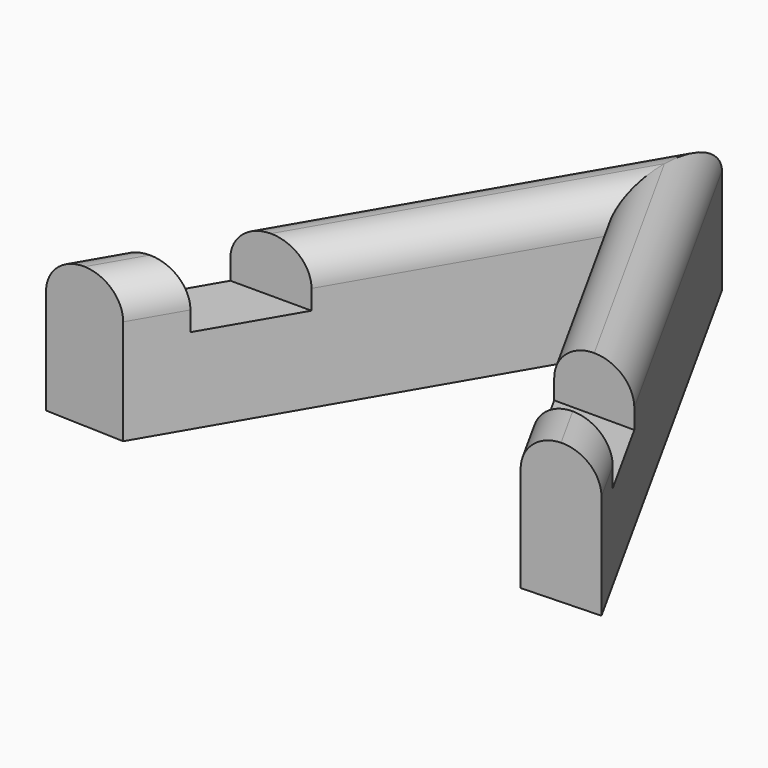
from build123d import *

# Parameters (mm, degrees)
F1_DEPTH = 10
F2_W     = 48.9705931395
F2_H     = 6.2394971028
F3_DEPTH = 3.9
F4_R     = 2.49999


# Not quite as in the source:
# - a fillet or chamfer is up to 0.001 mm smaller than in the source, because OpenCascade refuses the exact size


with BuildPart() as f1:
    # F0 (on Top) → F1 (new body)
    with BuildSketch(Plane.XY):
        Polygon((-14.5670969574, -24.9256566167), (0, 0), (13.7898046523, -24.9256566167), (19.3909112023, -24.7212815966), (0.1191440202, 10.1132547357), (-20.2359139567, -24.7161410615), align=None)
    extrude(amount=F1_DEPTH)

    # F2 (on face) → F3 (cut)
    with BuildSketch(Plane.XY.offset(10)):
        with Locations((2.1743709221, -18.3403375559)):
            Rectangle(F2_W, F2_H)
    extrude(amount=-F3_DEPTH, mode=Mode.SUBTRACT)

    # F4 (radius 2.5 in the source; OpenCascade refuses exactly that, so slightly less here)
    f4_edges = [f1.edges().sort_by_distance(p)[0] for p in [
        (-7.283681, -2.553667, 10),
        (7.126959, -2.553667, 10),
        (-4.447622, -7.610295, 10),
        (4.210299, -7.610295, 10),
        (-19.284459, -23.088114, 10),
        (-13.554419, -23.192871, 10),
        (12.831163, -23.192871, 10),
        (18.488804, -23.090684, 10),
    ]]
    fillet(f4_edges, radius=F4_R)


solid = f1.part
